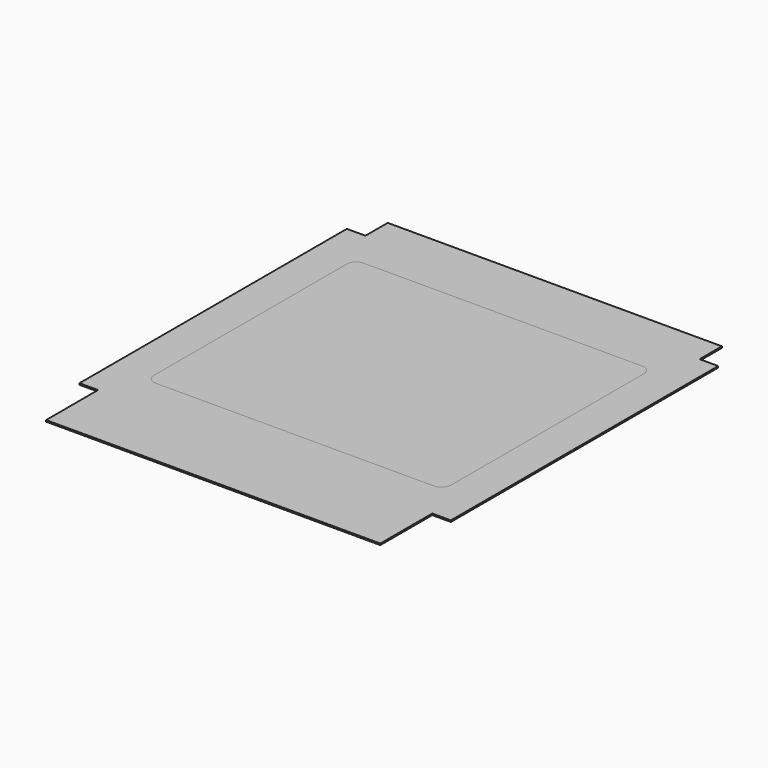
from build123d import *

# Parameters (mm, degrees)
F1_DEPTH = 1.5875
F2_DEPTH = 1.5875


# Not quite as in the source:
# - a length typed as a fraction of an inch, garbled in the dataset ("3 / 203.2 mm" for 3/8 in), is restored


with BuildPart() as f1:
    # F0 (on Top) → F1 (new body)
    with BuildSketch(Plane.XY):
        Polygon((-200, 180), (-200, -180), (-180, -180), (-180, -250), (0, -250), (180, -250), (180, -180), (200, -180), (200, 180), (180, 180), (180, 210), (0, 210), (-180, 210), (-180, 180), align=None)
        with BuildLine():
            Line((150, -140), (0, -140))
            Line((0, -140), (-150, -140))
            ThreePointArc((-150, -140), (-157.0710678119, -137.0710678119), (-160, -130))
            Line((-160, -130), (-160, 130))
            ThreePointArc((-160, 130), (-157.0710678119, 137.0710678119), (-150, 140))
            Line((-150, 140), (0, 140))
            Line((0, 140), (150, 140))
            ThreePointArc((150, 140), (157.0710678119, 137.0710678119), (160, 130))
            Line((160, 130), (160, -130))
            ThreePointArc((160, -130), (157.0710678119, -137.0710678119), (150, -140))
        make_face(mode=Mode.SUBTRACT)
    extrude(amount=F1_DEPTH)


with BuildPart() as f2:
    # F0 (on Top) → F2 (new body)
    with BuildSketch(Plane.XY):
        with BuildLine():
            Line((-150, -140), (0, -140))
            Line((0, -140), (150, -140))
            ThreePointArc((150, -140), (157.0710678119, -137.0710678119), (160, -130))
            Line((160, -130), (160, 130))
            ThreePointArc((160, 130), (157.0710678119, 137.0710678119), (150, 140))
            Line((150, 140), (0, 140))
            Line((0, 140), (-150, 140))
            ThreePointArc((-150, 140), (-157.0710678119, 137.0710678119), (-160, 130))
            Line((-160, 130), (-160, -130))
            ThreePointArc((-160, -130), (-157.0710678119, -137.0710678119), (-150, -140))
        make_face()
    extrude(amount=F2_DEPTH)


solid = Compound([f1.part, f2.part])
